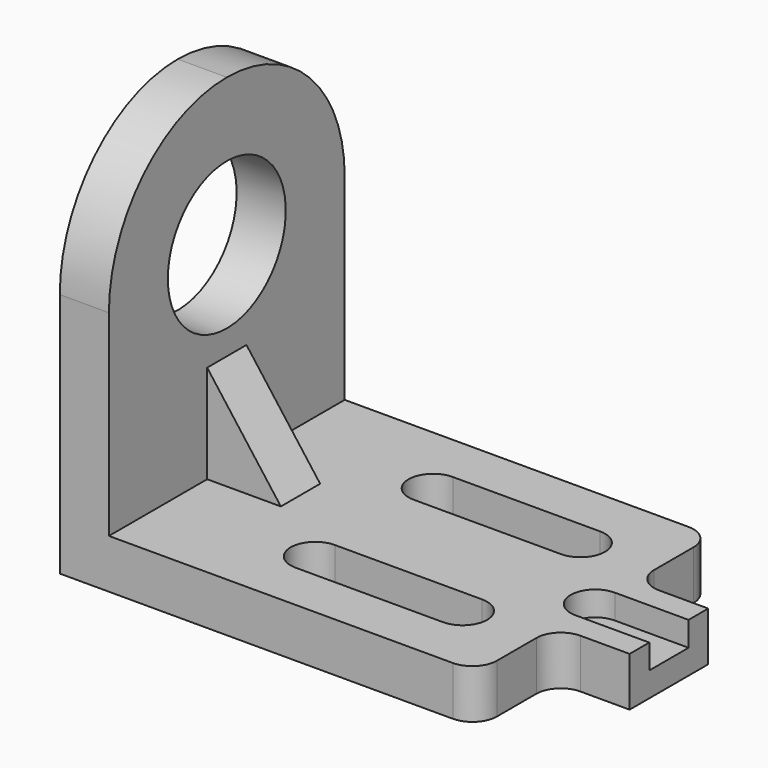
from build123d import *

# Parameters (mm, degrees)
F1_DEPTH  = 76.2
F3_DEPTH  = 12.7
F2_W      = 38.1
F2_H      = 50.8
F4_DEPTH  = 25.4
F5_DEPTH  = 25.4
F6_R      = 12.7
F7_R      = 38.1
F8_DEPTH  = 25.4
F9_DEPTH  = 25.401
F10_DEPTH = 12.7


# Not quite as in the source:
# - a pattern or mirror of a feature is missing from the dataset's text; its kind, count and spacing are read off the source's solid
# - a feature names something its author has since deleted; it is built from what else it names


with BuildPart() as f1:
    # F0 (on Front) → F1 (new body, symmetric)
    with BuildSketch(Plane.XZ):
        Polygon((25.4, 203.2), (0, 203.2), (0, 0), (254, 0), (254, 12.7), (254, 25.4), (63.5, 25.4), (25.4, 25.4), (25.4, 76.2), align=None)
    extrude(amount=F1_DEPTH, both=True)

    # F2 (on face) → F3 (cut)
    with BuildSketch(Plane.XY.offset(25.4)):
        with BuildLine():
            Line((215.9, -12.7), (254, -12.7))
            Line((254, -12.7), (254, 12.7))
            Line((254, 12.7), (215.9, 12.7))
            ThreePointArc((215.9, 12.7), (203.2, 0), (215.9, -12.7))
        make_face()
    extrude(amount=-F3_DEPTH, mode=Mode.SUBTRACT)

    # F2 (on face) → F4 (join)
    with BuildSketch(Plane.XY.offset(25.4)):
        with BuildLine():
            Line((25.4, -76.2), (215.9, -76.2))
            Line((215.9, -76.2), (215.9, -25.4))
            Line((215.9, -25.4), (254, -25.4))
            Line((254, -25.4), (254, -12.7))
            Line((254, -12.7), (215.9, -12.7))
            ThreePointArc((215.9, -12.7), (203.2, 0), (215.9, 12.7))
            Line((215.9, 12.7), (254, 12.7))
            Line((254, 12.7), (254, 25.4))
            Line((254, 25.4), (215.9, 25.4))
            Line((215.9, 25.4), (215.9, 76.2))
            Line((215.9, 76.2), (25.4, 76.2))
            Line((25.4, 76.2), (25.4, -76.2))
        make_face()
        with BuildLine():
            ThreePointArc((177.8, -25.4), (190.5, -38.1), (177.8, -50.8))
            Line((177.8, -50.8), (101.6, -50.8))
            ThreePointArc((101.6, -50.8), (88.9, -38.1), (101.6, -25.4))
            Line((101.6, -25.4), (177.8, -25.4))
        make_face(mode=Mode.SUBTRACT)
        with Locations((234.95, -50.8)):
            Rectangle(F2_W, F2_H)
        with BuildLine():
            Line((101.6, -50.8), (177.8, -50.8))
            ThreePointArc((177.8, -50.8), (190.5, -38.1), (177.8, -25.4))
            Line((177.8, -25.4), (101.6, -25.4))
            ThreePointArc((101.6, -25.4), (88.9, -38.1), (101.6, -50.8))
        make_face()
    extrude(amount=-F4_DEPTH)

    # F2 (on face) → F5 (cut)
    with BuildSketch(Plane.XY.offset(25.4)):
        with Locations((234.95, -50.8)):
            Rectangle(F2_W, F2_H)
        with Locations((234.95, 50.8)):
            Rectangle(F2_W, F2_H)
    extrude(amount=-F5_DEPTH, mode=Mode.SUBTRACT)

    # F6
    f6_edges = [f1.edges().sort_by_distance(p)[0] for p in [
        (215.9, -25.4, 12.7),
        (215.9, -76.2, 12.7),
        (215.9, 25.4, 12.7),
        (215.9, 76.2, 12.7),
    ]]
    fillet(f6_edges, radius=F6_R)

    # F7 (on face) → F8 (cut)
    with BuildSketch(Plane(origin=(0, 0, 0), x_dir=(0, -1, 0), z_dir=(-1, 0, 0))):
        with BuildLine():
            ThreePointArc((3.576e-07, 203.2), (53.8815368528, 180.8815366), (76.2, 127))
            Line((76.2, 127), (76.2, 203.2))
            Line((76.2, 203.2), (3.576e-07, 203.2))
        make_face()
        with Locations((0, 127)):
            Circle(F7_R)
        with BuildLine():
            ThreePointArc((-76.2, 127), (-53.8815366, 180.8815368528), (3.576e-07, 203.2))
            Line((3.576e-07, 203.2), (-76.2, 203.2))
            Line((-76.2, 203.2), (-76.2, 127))
        make_face()
    extrude(amount=-F8_DEPTH, mode=Mode.SUBTRACT)

    # F2 (on face) → F9 (cut, through all)
    with BuildSketch(Plane.XY.offset(25.4)):
        with BuildLine():
            Line((101.6, -50.8), (177.8, -50.8))
            ThreePointArc((177.8, -50.8), (190.5, -38.1), (177.8, -25.4))
            Line((177.8, -25.4), (101.6, -25.4))
            ThreePointArc((101.6, -25.4), (88.9, -38.1), (101.6, -50.8))
        make_face()
    f9 = extrude(amount=-F9_DEPTH, mode=Mode.SUBTRACT)

    # F9_copies: F9 across plane
    add(f9.mirror(Plane.ZX), mode=Mode.SUBTRACT)

    # F0 (on Front) → F10 (join, symmetric)
    with BuildSketch(Plane.XZ):
        Polygon((63.5, 25.4), (25.4, 76.2), (25.4, 25.4), align=None)
    extrude(amount=F10_DEPTH, both=True)


solid = f1.part
